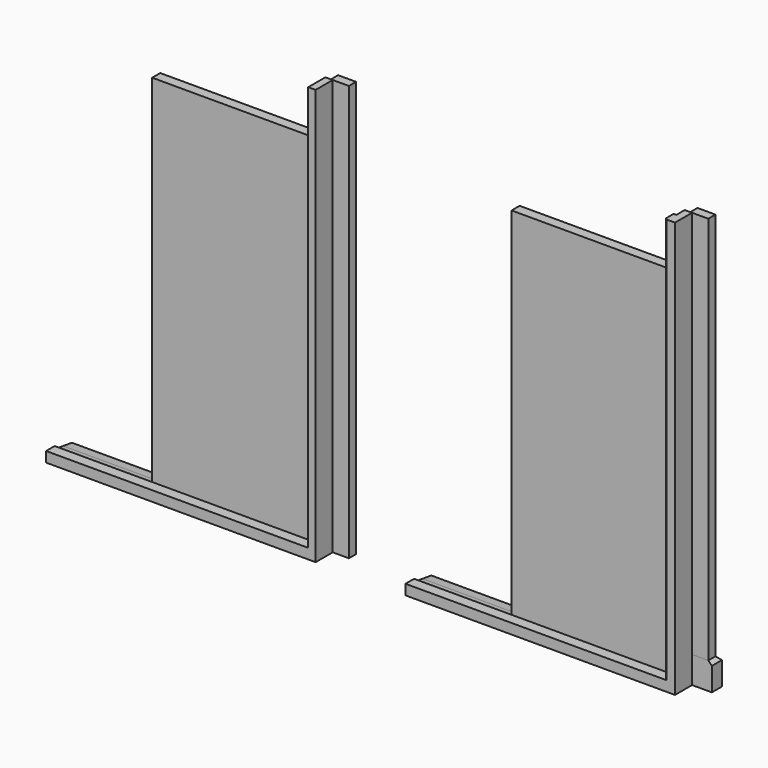
from build123d import *

# Parameters (mm, degrees)
F1_DEPTH  = 1500
F2_DEPTH  = 56
F4_DEPTH  = 3
F5_DEPTH  = 900
F7_DEPTH  = 2314.1348951653
F9_DEPTH  = 150
F10_W     = 120
F10_H     = 70
F11_DEPTH = 150
F12_SIZE  = 20
F13_R     = 5
F13_2_R   = 5
F14_DEPTH = 15
F15_DEPTH = 15
F16_DEPTH = 15
F17_DEPTH = 15
F19_DEPTH = 2257.1348951653


# Not quite as in the source:
# - a feature of the source that left no trace in its solid (it failed there, or was rolled back) is left out


with BuildPart() as f1:
    # F0 (on Right) → F1 (new body)
    with BuildSketch(Plane.YZ):
        Polygon((-183, 0), (0, 0), (0, 24), (-64, 33.3658536585), (-123, 42), (-123, 57), (-183, 57), align=None)
    extrude(amount=-F1_DEPTH)

    # F0 (on Right) → F2 (join)
    with BuildSketch(Plane.YZ):
        Polygon((-183, 161.9052439928), (-183, 57), (-123, 57), (-123, 42), (-64, 33.3658536585), (-64, 167.0590639114), (-64, 2314.1348951653), (-183, 2314.1348951653), align=None)
        Polygon((-65, 2037.5547998742), (-65, 37.5547998742), (-121, 45.7499218254), (-121, 2037.5547998742), align=None, mode=Mode.SUBTRACT)
        Polygon((-121, 45.7499218254), (-65, 37.5547998742), (-65, 2037.5547998742), (-121, 2037.5547998742), align=None)
    extrude(amount=-F2_DEPTH)


with BuildPart() as f4:
    # F3 (on face) → F4 (new body)
    with BuildSketch(Plane(origin=(-56, 0, 0), x_dir=(0, -1, 0), z_dir=(-1, 0, 0))):
        Polygon((65, 37.5920394199), (121, 45.5200997288), (121, 2036.7051838202), (65, 2036.7051838202), align=None)
    extrude(amount=F4_DEPTH)


with BuildPart() as f5:
    # F5 (new): a face of the model
    f5_faces = [f4.part.faces().sort_by_distance(p)[0] for p in [
        (-59, -92.9814562157, 1039.1293140523),
    ]]
    extrude(f5_faces, amount=F5_DEPTH)


with BuildPart() as f7:
    # F6 (on face) → F7 (new body, through all)
    with BuildSketch(Plane.XY.offset(2314.1348951653)):
        Polygon((-10, -14), (-10, -64), (0, -64), (90, -64), (90, -14), align=None)
    extrude(amount=-F7_DEPTH)


with BuildPart() as f8_1:
    # F8: copy of F7
    add(f7.part.moved(Location((2000, 0, 0))))


with BuildPart() as f8_2:
    # F8: copy of F1
    add(f1.part.moved(Location((2000, 0, 0))))


with BuildPart() as f8_3:
    # F8: copy of F5
    add(f5.part.moved(Location((2000, 0, 0))))

    # F17 (add): a face of the model
    f17_faces = [f8_3.faces().sort_by_distance(p)[0] for p in [
        (1941, -92.9814562157, 1039.1293140523),
    ]]
    extrude(f17_faces, amount=F17_DEPTH)


with BuildPart() as f9_tool:
    # F9 (cut): a face of the model
    f9_faces = [f8_1.part.faces().sort_by_distance(p)[0] for p in [
        (2040, -39, 0),
    ]]
    extrude(f9_faces, amount=-F9_DEPTH)


with BuildPart() as f8_1_1:
    add(f8_1.part)

    # F9: cut by f9_tool
    add(f9_tool.part, mode=Mode.SUBTRACT)


with BuildPart() as f8_2_1:
    add(f8_2.part)

    # F9: cut by f9_tool
    add(f9_tool.part, mode=Mode.SUBTRACT)

    # F13#2
    f13_2_edges = [f8_2_1.edges().sort_by_distance(p)[0] for p in [
        (1250, 0, 24),
    ]]
    fillet(f13_2_edges, radius=F13_2_R)

    # F16 (cut): a face of the model
    f16_faces = [f8_2_1.faces().sort_by_distance(p)[0] for p in [
        (1944, -123.3639578476, 1180.7575057396),
    ]]
    extrude(f16_faces, amount=-F16_DEPTH, mode=Mode.SUBTRACT)

    # F18 (on face) → F19 (join, through all)
    with BuildSketch(Plane.XY.offset(2314.1348951653)):
        with BuildLine():
            Line((1951.5, -183), (1959, -183))
            Line((1959, -183), (1959, -123))
            Line((1959, -123), (1944, -123))
            Line((1944, -123), (1944, -175.5))
            Line((1944, -175.5), (1946.5, -175.5))
            ThreePointArc((1946.5, -175.5), (1947.9644660941, -179.0355339059), (1951.5, -180.5))
            Line((1951.5, -180.5), (1951.5, -183))
        make_face()
    extrude(amount=-F19_DEPTH)


with BuildPart() as f11:
    # F10 (on face) → F11 (new body)
    with BuildSketch(Plane(origin=(0, 0, 150), x_dir=(1, 0, 0), z_dir=(0, 0, -1))):
        with Locations((2050, 29)):
            Rectangle(F10_W, F10_H)
    extrude(amount=F11_DEPTH)

    # F12
    f12_edges = [f11.edges().sort_by_distance(p)[0] for p in [
        (2050, 6, 150),
        (2110, -29, 150),
    ]]
    chamfer(f12_edges, length=F12_SIZE)


with BuildPart() as f1_1:
    add(f1.part)

    # F13
    f13_edges = [f1_1.edges().sort_by_distance(p)[0] for p in [
        (-750, 0, 24),
    ]]
    fillet(f13_edges, radius=F13_R)

    # F14 (cut): a face of the model
    f14_faces = [f1_1.faces().sort_by_distance(p)[0] for p in [
        (-56, -123.3639578476, 1180.7575057396),
    ]]
    extrude(f14_faces, amount=-F14_DEPTH, mode=Mode.SUBTRACT)


with BuildPart() as f4_1:
    add(f4.part)

    # F15 (add): a face of the model
    f15_faces = [f5.part.faces().sort_by_distance(p)[0] for p in [
        (-59, -92.9814562157, 1039.1293140523),
    ]]

    add(f5.part)  # F15 merges F5
    extrude(f15_faces, amount=F15_DEPTH)


solid = Compound([f7.part, f8_3.part, f8_1_1.part, f8_2_1.part, f11.part, f1_1.part, f4_1.part])
